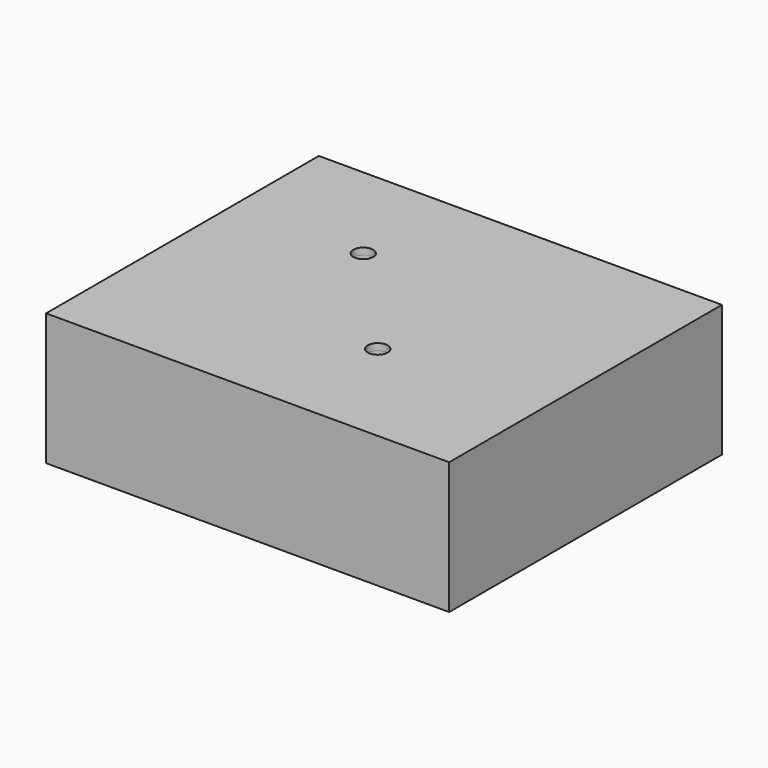
from build123d import *

# Parameters (mm, degrees)
F0_W     = 61.1153859645
F0_H     = 51.6923125833
F1_DEPTH = 20
F2_W     = 57.1153859645
F2_H     = 47.6923125833
F3_DEPTH = 19
F4_R     = 2.5
F4_R_2   = 1.5
F5_DEPTH = 10
F6_DEPTH = 1


# Not quite as in the source:
# - a feature of the source that left no trace in its solid (it failed there, or was rolled back) is left out


with BuildPart() as f1:
    # F0 (on Top) → F1 (new body)
    with BuildSketch(Plane.XY):
        with Locations((-0.1346161589, -0.9423075244)):
            Rectangle(F0_W, F0_H)
    extrude(amount=F1_DEPTH)

    # F2 (on face) → F3 (cut)
    with BuildSketch(Plane(origin=(0, 0, 0), x_dir=(1, 0, 0), z_dir=(0, 0, -1))):
        with Locations((-0.1346161589, 0.9423075244)):
            Rectangle(F2_W, F2_H)
    extrude(amount=-F3_DEPTH, mode=Mode.SUBTRACT)

    # F4 (on face) → F5 (join)
    with BuildSketch(Plane(origin=(0, 0, 19), x_dir=(1, 0, 0), z_dir=(0, 0, -1))):
        with Locations((-10.9730726108, -8.6767822504)):
            Circle(F4_R)
        with Locations((-10.9730726108, -8.6767822504)):
            Circle(F4_R_2, mode=Mode.SUBTRACT)
        with Locations((5.6683224998, 9.3844144205)):
            Circle(F4_R)
        with Locations((5.6683224998, 9.3844144205)):
            Circle(F4_R_2, mode=Mode.SUBTRACT)
    extrude(amount=F5_DEPTH)

    # F6 (cut): faces of the model
    f6_faces = [f1.faces().sort_by_distance(p)[0] for p in [
        (-10.9730726108, 8.6767822504, 19),
        (5.6683224998, -9.3844144205, 19),
    ]]
    extrude(f6_faces, amount=-F6_DEPTH, mode=Mode.SUBTRACT)


solid = f1.part
